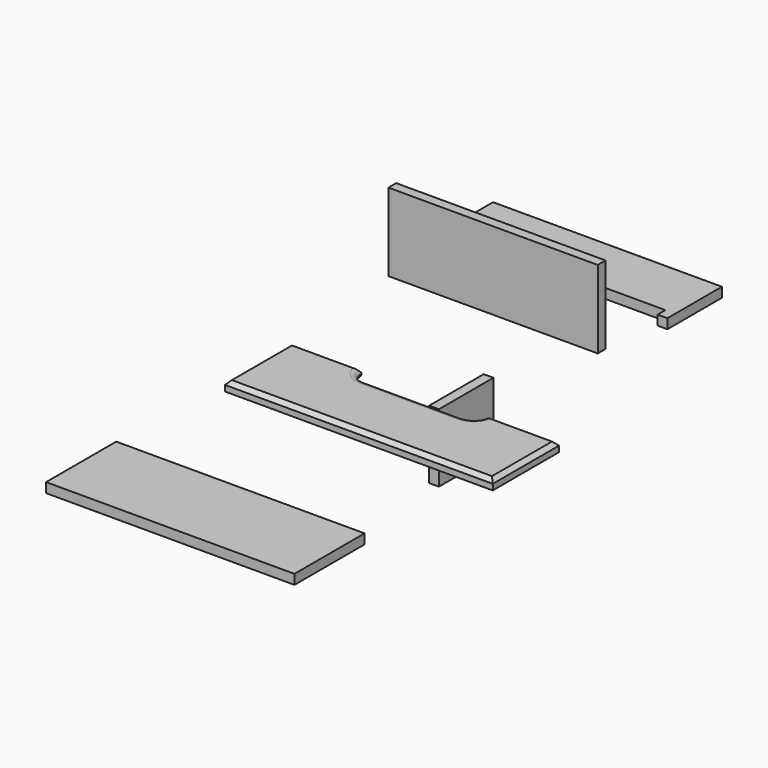
from build123d import *

# Parameters (mm, degrees)
F0_W         = 273.05
F0_H         = 101.6
F1_DEPTH     = 12.7
F3_DEPTH     = 12.7
F4_W         = 88.9
F4_H         = 88.9
F5_DEPTH     = 12.7
F7_DEPTH     = 12.7
F8_T1_DEPTH  = 127
F8_T4_ANGLE  = 147.318795695
F8_T6_ANGLE  = 147.318795695
F8_T8_ANGLE  = 147.318795695
F8_T10_ANGLE = 147.318795695
F9_T1_DEPTH  = 110.5832991577
F9_T3_DEPTH  = 134.0782991577
F9_T5_DEPTH  = 375.3782991577
F9_T7_DEPTH  = 110.5832991577
F10_W        = 323.85
F10_H        = 114.3
F11_DEPTH    = 12.7


# Not quite as in the source:
# - a fillet or chamfer that OpenCascade refuses, or shapes differently, is made with other operations: its cross-section is extruded or revolved along the edge and cut away or added


with BuildPart() as f1:
    # F0 (on Front) → F1 (new body)
    with BuildSketch(Plane.XZ):
        with Locations((2.9736794531, 50.4609997191)):
            Rectangle(F0_W, F0_H)
    extrude(amount=F1_DEPTH)


with BuildPart() as f3:
    # F2 (on Top) → F3 (new body)
    with BuildSketch(Plane.XY):
        Polygon((161.9328741789, 161.6237761021), (-136.5171258211, 161.6237761021), (-136.5171258211, 85.4237761021), (-136.5171258211, 72.7237761021), (-123.8171258211, 72.7237761021), (-123.8171258211, 85.4237761021), (149.2328741789, 85.4237761021), (149.2328741789, 72.7237761021), (161.9328741789, 72.7237761021), (161.9328741789, 85.4237761021), align=None)
    extrude(amount=F3_DEPTH)


with BuildPart() as f5:
    # F4 (on Right) → F5 (new body)
    with BuildSketch(Plane.YZ):
        with Locations((-68.700975406, -109.2356368899)):
            Rectangle(F4_W, F4_H)
    extrude(amount=F5_DEPTH)


with BuildPart() as f7:
    # F6 (on Top) → F7 (new body)
    with BuildSketch(Plane.XY):
        with BuildLine():
            Line((-12.0397317886, -207.9394155827), (-104.1147317886, -207.9394155827))
            Line((-104.1147317886, -207.9394155827), (-104.1147317886, -315.8894155827))
            Line((-104.1147317886, -315.8894155827), (245.1352682114, -315.8894155827))
            Line((245.1352682114, -315.8894155827), (245.1352682114, -207.9394155827))
            Line((245.1352682114, -207.9394155827), (153.0602682114, -207.9394155827))
            ThreePointArc((153.0602682114, -207.9394155827), (147.480652393, -221.4097997643), (134.0102682114, -226.9894155827))
            Line((134.0102682114, -226.9894155827), (7.0102682114, -226.9894155827))
            ThreePointArc((7.0102682114, -226.9894155827), (-6.4601159702, -221.4097997643), (-12.0397317886, -207.9394155827))
        make_face()
    extrude(amount=F7_DEPTH)

    # F8: fillet of radius 7.62 on 6 edges, made by hand

    # F8_s2 → F8_t1 (cut)
    with BuildSketch(Plane.YZ.offset(7.0102682114)):
        with BuildLine():
            ThreePointArc((-226.9894155827, 5.08), (-229.22126191, 10.4681536726), (-234.6094155827, 12.7))
            Line((-234.6094155827, 12.7), (-226.9894155827, 12.7))
            Line((-226.9894155827, 12.7), (-226.9894155827, 5.08))
        make_face()
        with BuildLine():
            ThreePointArc((-226.9894155827, 7.62), (-229.22126191, 2.2318463274), (-234.6094155827, 0))
            Line((-234.6094155827, 0), (-226.9894155827, 0))
            Line((-226.9894155827, 0), (-226.9894155827, 7.62))
        make_face()
    extrude(amount=F8_T1_DEPTH, mode=Mode.SUBTRACT)

    # F8_s3 → F8_t4 (revolve, cut)
    with BuildSketch(Plane(origin=(189.4426460264, -121.5322762083, 0), x_dir=(0, 0, 1), z_dir=(-0.8416879608, 0.5399642365, 0))):
        with BuildLine():
            ThreePointArc((7.62, -83.6093505), (2.2318463274, -81.3775041726), (0, -75.9893505))
            Line((0, -75.9893505), (0, -83.6093505))
            Line((0, -83.6093505), (7.62, -83.6093505))
        make_face()
    revolve(axis=Axis((134.0102682114, -207.9394155827, 0), (0, 0, -1)), revolution_arc=F8_T4_ANGLE, mode=Mode.SUBTRACT)

    # F8_s5 → F8_t6 (revolve, cut)
    with BuildSketch(Plane(origin=(189.4426460264, -121.5322762083, 0), x_dir=(0, 0, 1), z_dir=(-0.8416879608, 0.5399642365, 0))):
        with BuildLine():
            ThreePointArc((5.08, -83.6093505), (10.4681536726, -81.3775041726), (12.7, -75.9893505))
            Line((12.7, -75.9893505), (12.7, -83.6093505))
            Line((12.7, -83.6093505), (5.08, -83.6093505))
        make_face()
    revolve(axis=Axis((134.0102682114, -207.9394155827, 12.7), (0, 0, -1)), revolution_arc=F8_T6_ANGLE, mode=Mode.SUBTRACT)

    # F8_s7 → F8_t8 (revolve, cut)
    with BuildSketch(Plane.YZ.offset(7.0102682114)):
        with BuildLine():
            ThreePointArc((-226.9894155827, 7.62), (-229.22126191, 2.2318463274), (-234.6094155827, 0))
            Line((-234.6094155827, 0), (-226.9894155827, 0))
            Line((-226.9894155827, 0), (-226.9894155827, 7.62))
        make_face()
    revolve(axis=Axis((7.0102682114, -207.9394155827, 0), (0, 0, -1)), revolution_arc=F8_T8_ANGLE, mode=Mode.SUBTRACT)

    # F8_s9 → F8_t10 (revolve, cut)
    with BuildSketch(Plane.YZ.offset(7.0102682114)):
        with BuildLine():
            ThreePointArc((-226.9894155827, 5.08), (-229.22126191, 10.4681536726), (-234.6094155827, 12.7))
            Line((-234.6094155827, 12.7), (-226.9894155827, 12.7))
            Line((-226.9894155827, 12.7), (-226.9894155827, 5.08))
        make_face()
    revolve(axis=Axis((7.0102682114, -207.9394155827, 12.7), (0, 0, -1)), revolution_arc=F8_T10_ANGLE, mode=Mode.SUBTRACT)

    # F9: chamfer of 5.08 on 5 edges, made by hand

    # F9_s2 → F9_t1 (cut)
    with BuildSketch(Plane.YZ.offset(-117.1788813675)):
        Polygon((-213.0194155827, 12.7), (-207.9394155827, 7.62), (-207.9394155827, 12.7), align=None)
    extrude(amount=F9_T1_DEPTH, mode=Mode.SUBTRACT)

    # F9_s4 → F9_t3 (cut)
    with BuildSketch(Plane.XZ.offset(194.8752660038)):
        Polygon((-99.0347317886, 12.7), (-104.1147317886, 7.62), (-104.1147317886, 12.7), align=None)
        Polygon((240.0552682114, 12.7), (245.1352682114, 7.62), (245.1352682114, 12.7), align=None)
    extrude(amount=F9_T3_DEPTH, mode=Mode.SUBTRACT)

    # F9_s6 → F9_t5 (cut)
    with BuildSketch(Plane.YZ.offset(-117.1788813675)):
        Polygon((-310.8094155827, 12.7), (-315.8894155827, 7.62), (-315.8894155827, 12.7), align=None)
    extrude(amount=F9_T5_DEPTH, mode=Mode.SUBTRACT)

    # F9_s8 → F9_t7 (cut)
    with BuildSketch(Plane.YZ.offset(147.6161186325)):
        Polygon((-207.9394155827, 7.62), (-213.0194155827, 12.7), (-207.9394155827, 12.7), align=None)
    extrude(amount=F9_T7_DEPTH, mode=Mode.SUBTRACT)


with BuildPart() as f11:
    # F10 (on Top) → F11 (new body)
    with BuildSketch(Plane.XY):
        with Locations((55.6372515857, -547.4844523445)):
            Rectangle(F10_W, F10_H)
    extrude(amount=F11_DEPTH)


solid = Compound([f1.part, f3.part, f5.part, f7.part, f11.part])
